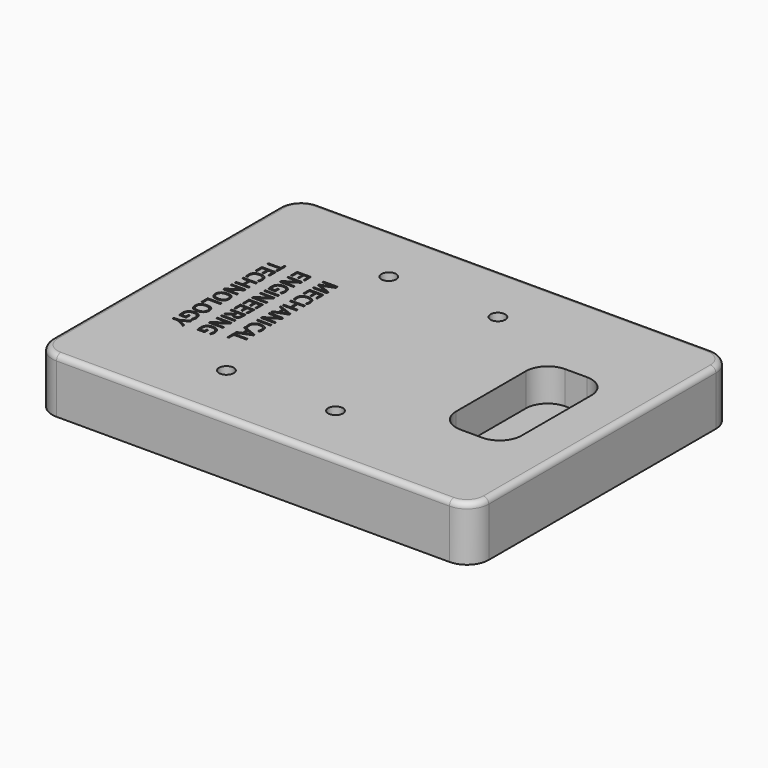
from build123d import *

# Parameters (mm, degrees)
F1_DEPTH       = 50
F2_R           = 20
F4_DEPTH       = 30
F6_D           = 13.5
F6_CBORE_D     = 26
F6_CBORE_DEPTH = 12
F7_TEXT_SIZE   = 17.9197928973
F8_DEPTH       = 2
F9_R           = 5


# Not quite as in the source:
# - Text() gives the source's letters only with a copy of the font that has no kerning and outlines rounded to 1/6400 em; it was checked with that copy


with BuildPart() as f1:
    # F0 (on Top) → F1 (new body)
    with BuildSketch(Plane.XY):
        Polygon((200, 0), (0, 0), (-200, 0), (-200, -150), (200, -150), align=None)
        Polygon((-200, 0), (0, 0), (200, 0), (200, 150), (-200, 150), align=None)
    extrude(amount=F1_DEPTH)

    # F2
    f2_edges = [f1.edges().sort_by_distance(p)[0] for p in [
        (200, -150, 25),
        (200, 150, 25),
        (-200, 150, 25),
        (-200, -150, 25),
    ]]
    fillet(f2_edges, radius=F2_R)

    # F3 (on face) → F4 (cut)
    with BuildSketch(Plane.XY.offset(50)):
        with BuildLine():
            Line((98, 40), (98, 0))
            Line((98, 0), (98, -40))
            ThreePointArc((98, -40), (103.8578643763, -54.1421356237), (118, -60))
            Line((118, -60), (138, -60))
            ThreePointArc((138, -60), (152.1421356237, -54.1421356237), (158, -40))
            Line((158, -40), (158, 40))
            ThreePointArc((158, 40), (152.1421356237, 54.1421356237), (138, 60))
            Line((138, 60), (118, 60))
            ThreePointArc((118, 60), (103.8578643763, 54.1421356237), (98, 40))
        make_face()
    extrude(amount=-F4_DEPTH, mode=Mode.SUBTRACT)

    # F6 (through all)
    with Locations(Plane(origin=(0, 0, 0), x_dir=(1, 0, 0), z_dir=(0, 0, -1))):
        with Locations((-70, 93), (30, 93), (30, -93), (-70, -93)):
            CounterBoreHole(F6_D / 2, F6_CBORE_D / 2, F6_CBORE_DEPTH)

    # F7 (on face) → F8 (cut)
    with BuildSketch(Plane.XY.offset(50)):
        with Locations(Location((-101.5529623449, 59.6855102022), (0, 0, -90))):
            Text('MECHANICAL', F7_TEXT_SIZE, font='Open Sans', text_align=(TextAlign.LEFT, TextAlign.BOTTOM))
        with Locations(Location((-125.9238806852, 59.6855102022), (0, 0, -90))):
            Text('ENGINEERING', F7_TEXT_SIZE, font='Open Sans', text_align=(TextAlign.LEFT, TextAlign.BOTTOM))
        with Locations(Location((-150.2947990255, 59.6855102022), (0, 0, -90))):
            Text('TECHNOLOGY', F7_TEXT_SIZE, font='Open Sans', text_align=(TextAlign.LEFT, TextAlign.BOTTOM))
    extrude(amount=-F8_DEPTH, mode=Mode.SUBTRACT)

    # F9
    f9_edges = [f1.edges().sort_by_distance(p)[0] for p in [
        (-200, 0, 50),
    ]]
    fillet(f9_edges, radius=F9_R)


solid = f1.part
